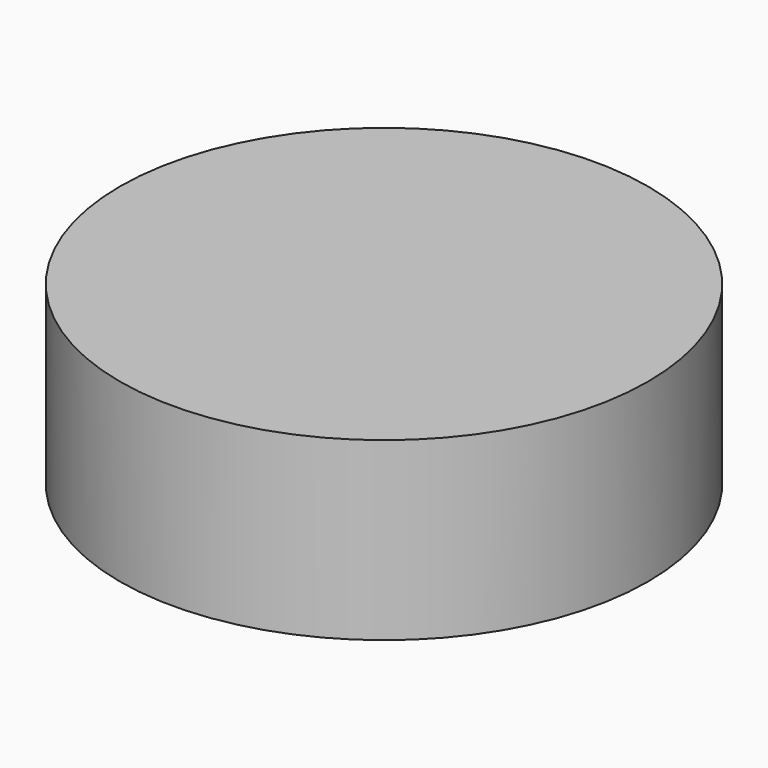
from build123d import *

# Parameters (mm, degrees)
F0_R         = 19.05
F1_DEPTH     = 12.7
F2_TEXT_SIZE = 32.4535835496
F3_DEPTH     = 2.54


# Not quite as in the source:
# - Text() gives the source's letters only with a copy of the font that has no kerning and outlines rounded to 1/6400 em; it was checked with that copy


with BuildPart() as f1:
    # F0 (on Top) → F1 (new body)
    with BuildSketch(Plane.XY):
        Circle(F0_R)
    extrude(amount=F1_DEPTH)

    # F2 (on Top) → F3 (cut)
    with BuildSketch(Plane.XY):
        with Locations((-12.7, -10.6665801557)):
            Text('Q', F2_TEXT_SIZE, font='Open Sans', text_align=(TextAlign.LEFT, TextAlign.BOTTOM))
    extrude(amount=F3_DEPTH, mode=Mode.SUBTRACT)


solid = f1.part
